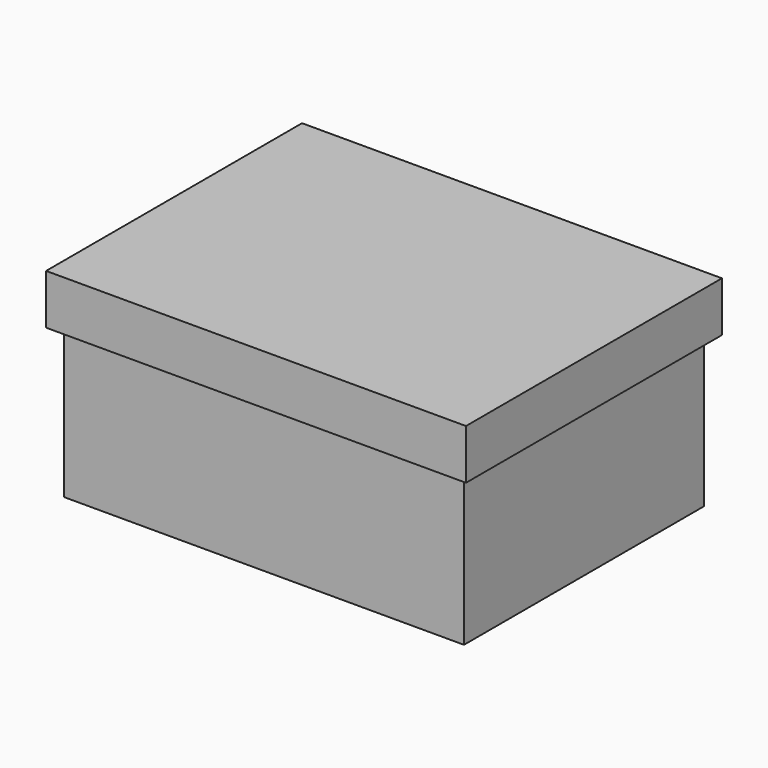
from build123d import *

# Parameters (mm, degrees)
F0_W     = 80
F0_H     = 60
F1_DEPTH = 40
F2_W     = 80
F2_H     = 10
F3_DEPTH = 2
F5_DEPTH = 2
F7_DEPTH = 2
F9_DEPTH = 2


with BuildPart() as f1:
    # F0 (on Top) → F1 (new body)
    with BuildSketch(Plane.XY):
        Rectangle(F0_W, F0_H)
    extrude(amount=F1_DEPTH)

    # F2 (on face) → F3 (join)
    with BuildSketch(Plane.XZ.offset(30)):
        with Locations((0, 35)):
            Rectangle(F2_W, F2_H)
    extrude(amount=F3_DEPTH)

    # F4 (on face) → F5 (join)
    with BuildSketch(Plane.YZ.offset(40)):
        Polygon((-32, 40), (-32, 30), (-30, 30), (30, 30), (30, 40), align=None)
    extrude(amount=F5_DEPTH)

    # F6 (on face) → F7 (join)
    with BuildSketch(Plane(origin=(0, 30, 0), x_dir=(-1, 0, 0), z_dir=(0, 1, 0))):
        Polygon((-42, 40), (-42, 30), (-40, 30), (40, 30), (40, 40), align=None)
    extrude(amount=F7_DEPTH)

    # F8 (on face) → F9 (join)
    with BuildSketch(Plane(origin=(-40, 0, 0), x_dir=(0, -1, 0), z_dir=(-1, 0, 0))):
        Polygon((-32, 40), (-32, 30), (-30, 30), (30, 30), (32, 30), (32, 40), align=None)
    extrude(amount=F9_DEPTH)


solid = f1.part
